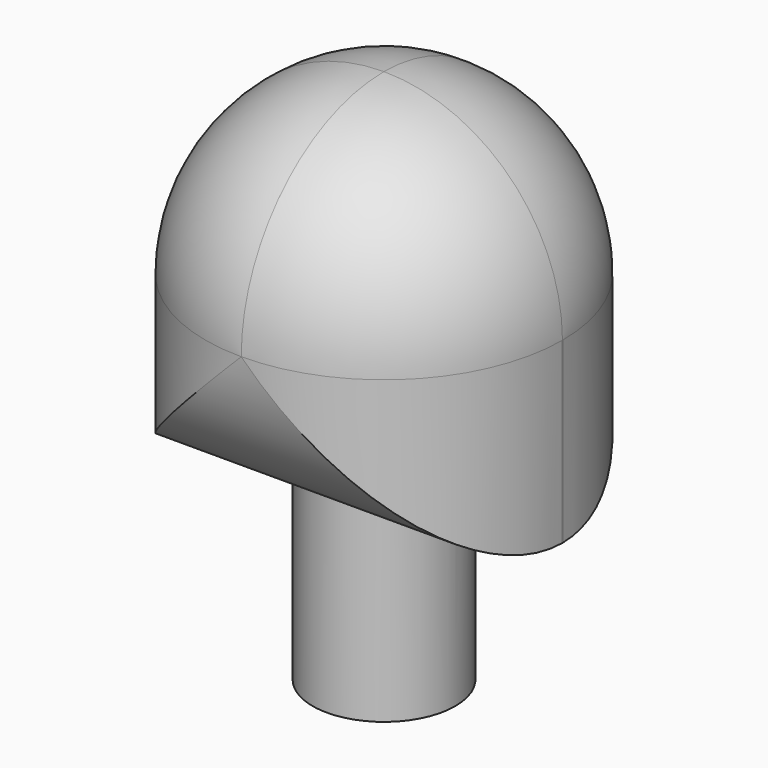
from build123d import *

# Parameters (mm, degrees)
F0_R         = 10
F1_DEPTH     = 25
F2_W         = 50
F2_H         = 50
F3_DEPTH     = 50
F4_T1_DEPTH  = 87.4998500005
F4_T3_DEPTH  = 0.0002
F4_T5_DEPTH  = 0.0002
F4_S9_W      = 25.5
F4_S9_H      = 25.5
F4_T10_DEPTH = 25.5
F4_S15_W     = 25.5
F4_S15_H     = 25.5
F4_T16_DEPTH = 25.5
F4_S21_W     = 25.5
F4_S21_H     = 25.5
F4_T22_DEPTH = 25.5
F4_S27_W     = 25.5
F4_S27_H     = 25.5
F4_T28_DEPTH = 25.5
F4_T34_DEPTH = 174.999500001
F4_S35_R     = 10
F4_T36_DEPTH = 91
F4_T40_DEPTH = 174.999500001
F4_S41_R     = 10
F4_T42_DEPTH = 91


# Not quite as in the source:
# - a fillet or chamfer that OpenCascade refuses, or shapes differently, is made with other operations: its cross-section is extruded or revolved along the edge and cut away or added


with BuildPart() as f1:
    # F0 (on Top) → F1 (new body)
    with BuildSketch(Plane.XY):
        Circle(F0_R)
    extrude(amount=F1_DEPTH)

    # F2 (on face) → F3 (join)
    with BuildSketch(Plane.XY.offset(25)):
        Rectangle(F2_W, F2_H)
    extrude(amount=F3_DEPTH)

    # F4: fillet of radius 25 on 10 edges, made by hand

    # F4_s2 → F4_t1 (cut)
    with BuildSketch(Plane.XY.offset(-37.4997500005)):
        with BuildLine():
            ThreePointArc((-0.0001, -25.0001), (-17.6777695297, -17.6777695297), (-25.0001, -0.0001))
            Line((-25.0001, -0.0001), (-25.5001, -0.0001))
            ThreePointArc((-25.5001, -0.0001), (-25.5, -12.50005), (-25.5, -25))
            Line((-25.5, -25), (-25, -25.5))
            ThreePointArc((-25, -25.5), (-12.50005, -25.5), (-0.0001, -25.5001))
            Line((-0.0001, -25.5001), (-0.0001, -25.0001))
        make_face()
        with BuildLine():
            ThreePointArc((25.0001, -0.0001), (17.6777695297, -17.6777695297), (0.0001, -25.0001))
            Line((0.0001, -25.0001), (0.0001, -25.5001))
            ThreePointArc((0.0001, -25.5001), (12.50005, -25.5), (25, -25.5))
            Line((25, -25.5), (25.5, -25))
            ThreePointArc((25.5, -25), (25.5, -12.50005), (25.5001, -0.0001))
            Line((25.5001, -0.0001), (25.0001, -0.0001))
        make_face()
        with BuildLine():
            ThreePointArc((25.0001, 0.0001), (17.6777695297, 17.6777695297), (0.0001, 25.0001))
            Line((0.0001, 25.0001), (0.0001, 25.5001))
            ThreePointArc((0.0001, 25.5001), (12.50005, 25.5), (25, 25.5))
            Line((25, 25.5), (25.5, 25))
            ThreePointArc((25.5, 25), (25.5, 12.50005), (25.5001, 0.0001))
            Line((25.5001, 0.0001), (25.0001, 0.0001))
        make_face()
        with BuildLine():
            ThreePointArc((-0.0001, 25.0001), (-17.6777695297, 17.6777695297), (-25.0001, 0.0001))
            Line((-25.0001, 0.0001), (-25.5001, 0.0001))
            ThreePointArc((-25.5001, 0.0001), (-25.5, 12.50005), (-25.5, 25))
            Line((-25.5, 25), (-25, 25.5))
            ThreePointArc((-25, 25.5), (-12.50005, 25.5), (-0.0001, 25.5001))
            Line((-0.0001, 25.5001), (-0.0001, 25.0001))
        make_face()
    extrude(amount=F4_T1_DEPTH, mode=Mode.SUBTRACT)

    # F4_s4 → F4_t3 (cut)
    with BuildSketch(Plane.YZ.offset(-0.0001)):
        with BuildLine():
            ThreePointArc((-25.0001, 50.0001), (-17.6777695297, 67.6777695297), (-0.0001, 75.0001))
            Line((-0.0001, 75.0001), (-0.0001, 75.5001))
            ThreePointArc((-0.0001, 75.5001), (-12.50005, 75.5), (-25, 75.5))
            Line((-25, 75.5), (-25.5, 75))
            ThreePointArc((-25.5, 75), (-25.5, 62.50005), (-25.5001, 50.0001))
            Line((-25.5001, 50.0001), (-25.0001, 50.0001))
        make_face()
        with BuildLine():
            ThreePointArc((25.0001, 50.0001), (17.6777695297, 67.6777695297), (0.0001, 75.0001))
            Line((0.0001, 75.0001), (0.0001, 75.5001))
            ThreePointArc((0.0001, 75.5001), (12.50005, 75.5), (25, 75.5))
            Line((25, 75.5), (25.5, 75))
            ThreePointArc((25.5, 75), (25.5, 62.50005), (25.5001, 50.0001))
            Line((25.5001, 50.0001), (25.0001, 50.0001))
        make_face()
    extrude(amount=F4_T3_DEPTH, mode=Mode.SUBTRACT)

    # F4_s6 → F4_t5 (cut)
    with BuildSketch(Plane.XZ.offset(-0.0001)):
        with BuildLine():
            ThreePointArc((25.0001, 50.0001), (17.6777695297, 67.6777695297), (0.0001, 75.0001))
            Line((0.0001, 75.0001), (0.0001, 75.5001))
            ThreePointArc((0.0001, 75.5001), (12.50005, 75.5), (25, 75.5))
            Line((25, 75.5), (25.5, 75))
            ThreePointArc((25.5, 75), (25.5, 62.50005), (25.5001, 50.0001))
            Line((25.5001, 50.0001), (25.0001, 50.0001))
        make_face()
        with BuildLine():
            ThreePointArc((-0.0001, 75.0001), (-17.6777695297, 67.6777695297), (-25.0001, 50.0001))
            Line((-25.0001, 50.0001), (-25.5001, 50.0001))
            ThreePointArc((-25.5001, 50.0001), (-25.5, 62.50005), (-25.5, 75))
            Line((-25.5, 75), (-25, 75.5))
            ThreePointArc((-25, 75.5), (-12.50005, 75.5), (-0.0001, 75.5001))
            Line((-0.0001, 75.5001), (-0.0001, 75.0001))
        make_face()
    extrude(amount=F4_T5_DEPTH, mode=Mode.SUBTRACT)


with BuildPart() as f4_tool8:
    # F4_s9 → F4_t10 (new body)
    with BuildSketch(Plane.XZ.offset(0.0001)):
        with Locations((-12.7501, 62.7501)):
            Rectangle(F4_S9_W, F4_S9_H)
    extrude(amount=F4_T10_DEPTH)

    # F4_s11 → F4_t12 (revolve, cut)
    with BuildSketch(Plane(origin=(-0.0001, -0.0001, 50.0001), x_dir=(0.7071067812, 0, -0.7071067812), z_dir=(-0.7071067812, 0, -0.7071067812))):
        with BuildLine():
            ThreePointArc((0, -25), (25, 0), (0, 25))
            Line((0, 25), (0, -25))
        make_face()
    revolve(axis=Axis((-0.0001, -0.0001, 50.0001), (0, -1, 0)), mode=Mode.SUBTRACT)


with BuildPart() as f1_1:
    add(f1.part)

    # F4_t7: cut F4_tool8
    add(f4_tool8.part, mode=Mode.SUBTRACT)


with BuildPart() as f4_tool14:
    # F4_s15 → F4_t16 (new body)
    with BuildSketch(Plane.YZ.offset(0.0001)):
        with Locations((-12.7501, 62.7501)):
            Rectangle(F4_S15_W, F4_S15_H)
    extrude(amount=F4_T16_DEPTH)

    # F4_s17 → F4_t18 (revolve, cut)
    with BuildSketch(Plane(origin=(0.0001, -0.0001, 50.0001), x_dir=(0, 0.7071067812, -0.7071067812), z_dir=(0, -0.7071067812, -0.7071067812))):
        with BuildLine():
            ThreePointArc((0, -25), (25, 0), (0, 25))
            Line((0, 25), (0, -25))
        make_face()
    revolve(axis=Axis((0.0001, -0.0001, 50.0001), (1, 0, 0)), mode=Mode.SUBTRACT)


with BuildPart() as f1_2:
    add(f1_1.part)

    # F4_t13: cut F4_tool14
    add(f4_tool14.part, mode=Mode.SUBTRACT)


with BuildPart() as f4_tool20:
    # F4_s21 → F4_t22 (new body)
    with BuildSketch(Plane.YZ.offset(0.0001)):
        with Locations((12.7501, 62.7501)):
            Rectangle(F4_S21_W, F4_S21_H)
    extrude(amount=F4_T22_DEPTH)

    # F4_s23 → F4_t24 (revolve, cut)
    with BuildSketch(Plane(origin=(0.0001, 0.0001, 50.0001), x_dir=(0, -0.7071067812, -0.7071067812), z_dir=(0, -0.7071067812, 0.7071067812))):
        with BuildLine():
            ThreePointArc((0, -25), (25, 0), (0, 25))
            Line((0, 25), (0, -25))
        make_face()
    revolve(axis=Axis((0.0001, 0.0001, 50.0001), (1, 0, 0)), mode=Mode.SUBTRACT)


with BuildPart() as f1_3:
    add(f1_2.part)

    # F4_t19: cut F4_tool20
    add(f4_tool20.part, mode=Mode.SUBTRACT)


with BuildPart() as f4_tool26:
    # F4_s27 → F4_t28 (new body)
    with BuildSketch(Plane.XZ.offset(-0.0001)):
        with Locations((-12.7501, 62.7501)):
            Rectangle(F4_S27_W, F4_S27_H)
    extrude(amount=-F4_T28_DEPTH)

    # F4_s29 → F4_t30 (revolve, cut)
    with BuildSketch(Plane(origin=(-0.0001, 0.0001, 50.0001), x_dir=(0.7071067812, 0, -0.7071067812), z_dir=(0.7071067812, 0, 0.7071067812))):
        with BuildLine():
            ThreePointArc((0, -25), (25, 0), (0, 25))
            Line((0, 25), (0, -25))
        make_face()
    revolve(axis=Axis((-0.0001, 0.0001, 50.0001), (0, 1, 0)), mode=Mode.SUBTRACT)


with BuildPart() as f1_4:
    add(f1_3.part)

    # F4_t25: cut F4_tool26
    add(f4_tool26.part, mode=Mode.SUBTRACT)


with BuildPart() as f4_tool32:
    # F4_s33 → F4_t34 (new body)
    with BuildSketch(Plane.YZ.offset(-87.4997500005)):
        with BuildLine():
            ThreePointArc((-25.0001, 49.9999), (-17.6777695297, 32.3222304703), (-0.0001, 24.9999))
            Line((-0.0001, 24.9999), (-0.0001, 24.4999))
            ThreePointArc((-0.0001, 24.4999), (-12.50005, 24.5), (-25, 24.5))
            Line((-25, 24.5), (-25.5, 25))
            ThreePointArc((-25.5, 25), (-25.5, 37.49995), (-25.5001, 49.9999))
            Line((-25.5001, 49.9999), (-25.0001, 49.9999))
        make_face()
    extrude(amount=F4_T34_DEPTH)

    # F4_s35 → F4_t36 (cut, symmetric)
    with BuildSketch(Plane.XY.offset(37.2)):
        Circle(F4_S35_R)
    extrude(amount=F4_T36_DEPTH, both=True, mode=Mode.SUBTRACT)


with BuildPart() as f1_5:
    add(f1_4.part)

    # F4_t31: cut F4_tool32
    add(f4_tool32.part, mode=Mode.SUBTRACT)


with BuildPart() as f4_tool38:
    # F4_s39 → F4_t40 (new body)
    with BuildSketch(Plane.YZ.offset(87.4997500005)):
        with BuildLine():
            ThreePointArc((25.0001, 49.9999), (17.6777695297, 32.3222304703), (0.0001, 24.9999))
            Line((0.0001, 24.9999), (0.0001, 24.4999))
            ThreePointArc((0.0001, 24.4999), (12.50005, 24.5), (25, 24.5))
            Line((25, 24.5), (25.5, 25))
            ThreePointArc((25.5, 25), (25.5, 37.49995), (25.5001, 49.9999))
            Line((25.5001, 49.9999), (25.0001, 49.9999))
        make_face()
    extrude(amount=-F4_T40_DEPTH)

    # F4_s41 → F4_t42 (cut, symmetric)
    with BuildSketch(Plane.XY.offset(37.2)):
        Circle(F4_S41_R)
    extrude(amount=F4_T42_DEPTH, both=True, mode=Mode.SUBTRACT)


with BuildPart() as f1_6:
    add(f1_5.part)

    # F4_t37: cut F4_tool38
    add(f4_tool38.part, mode=Mode.SUBTRACT)


solid = f1_6.part
